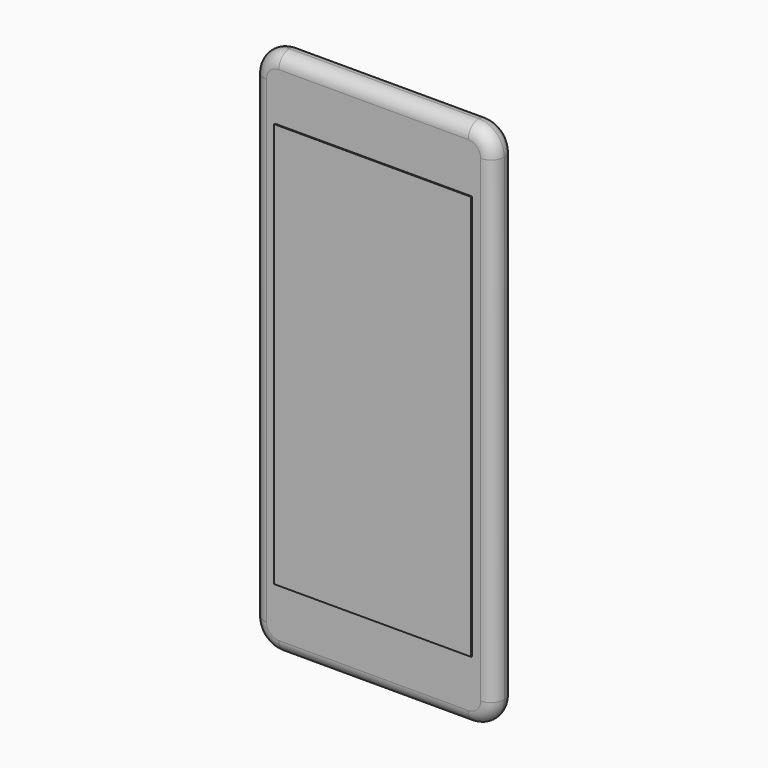
from build123d import *

# Parameters (mm, degrees)
F1_DEPTH = 6.5
F2_R     = 3.24999
F5_R     = 4.1935700789
F6_DEPTH = 0.254
F7_W     = 48.9017218351
F7_H     = 100.4664152861
F8_DEPTH = 0.254


# Not quite as in the source:
# - a fillet or chamfer is up to 0.001 mm smaller than in the source, because OpenCascade refuses the exact size
# - the program builds the solid bodies; features that only make, move or delete a surface that nothing else refers to are left out


with BuildPart() as f1:
    # F0 (on Front) → F1 (new body)
    with BuildSketch(Plane.XZ):
        with BuildLine():
            ThreePointArc((29.8388717587, 59.2516543508), (27.9789998192, 63.7417824113), (23.4888717587, 65.6016543508))
            Line((23.4888717587, 65.6016543508), (-23.4888717587, 65.6016543508))
            ThreePointArc((-23.4888717587, 65.6016543508), (-27.9789998192, 63.7417824113), (-29.8388717587, 59.2516543508))
            Line((-29.8388717587, 59.2516543508), (-29.8388717587, -59.2516543508))
            ThreePointArc((-29.8388717587, -59.2516543508), (-27.9789998192, -63.7417824113), (-23.4888717587, -65.6016543508))
            Line((-23.4888717587, -65.6016543508), (23.4888717587, -65.6016543508))
            ThreePointArc((23.4888717587, -65.6016543508), (27.9789998192, -63.7417824113), (29.8388717587, -59.2516543508))
            Line((29.8388717587, -59.2516543508), (29.8388717587, 59.2516543508))
        make_face()
    extrude(amount=F1_DEPTH)

    # F2 (radius 3.25 in the source; OpenCascade refuses exactly that, so slightly less here)
    f2_edges = [f1.edges().sort_by_distance(p)[0] for p in [
        (29.838872, 0, 0),
        (29.838872, -6.5, 0),
        (-29.838872, -6.5, 0),
        (0, 0, 65.601654),
        (0, -6.5, 65.601654),
        (-27.979, -6.5, 63.741782),
        (-27.979, 0, 63.741782),
        (27.979, -6.5, 63.741782),
        (27.979, 0, 63.741782),
        (27.979, -6.5, -63.741782),
        (0, -6.5, -65.601654),
        (-27.979, -6.5, -63.741782),
        (27.979, 0, -63.741782),
        (0, 0, -65.601654),
        (-27.979, 0, -63.741782),
        (-29.838872, -3.25, 59.251654),
        (-29.838872, -3.25, -59.251654),
        (-29.838872, 0, 0),
    ]]
    fillet(f2_edges, radius=F2_R)

    # F5 (on Front) → F6 (join)
    with BuildSketch(Plane.XZ):
        with Locations((0, -55.7777807117)):
            Circle(F5_R)
    extrude(amount=F6_DEPTH)

    # F7 (on face) → F8 (join)
    with BuildSketch(Plane.XZ.offset(6.5)):
        Rectangle(F7_W, F7_H)
    extrude(amount=F8_DEPTH)


solid = f1.part
